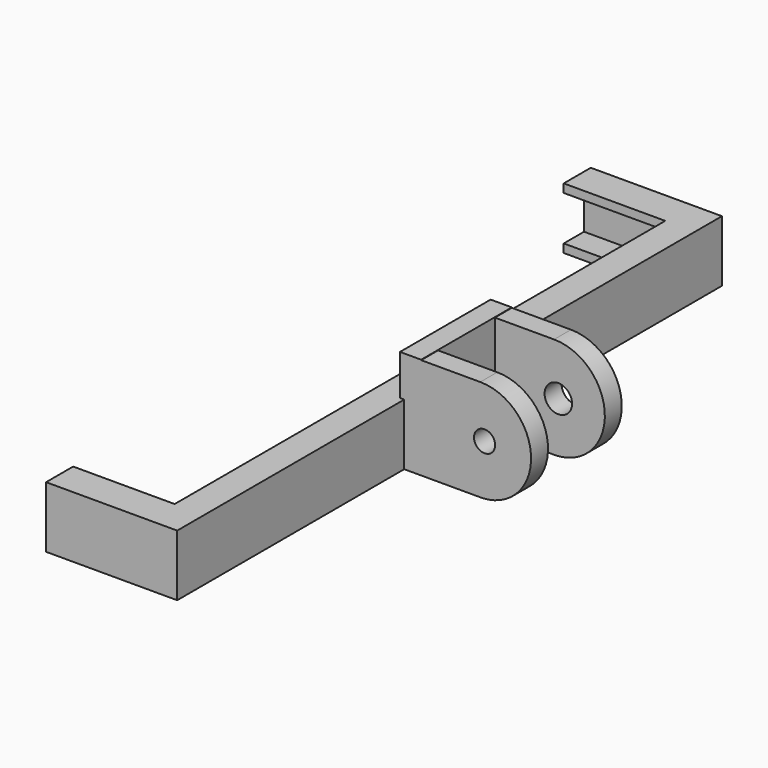
from build123d import *

# Parameters (mm, degrees)
F0_R          = 3.3
F0_R_2        = 2.5
F1_DEPTH      = 5
F2_DEPTH      = 5
F2_DEPTH_BACK = 21.8
F5_R          = 3.25
F5_R_2        = 2.5
F6_DEPTH      = 6
F7_W          = 59.1
F7_H          = 2
F7_W_2        = 6
F8_DEPTH      = 1
F7_W_3        = 13.4
F9_DEPTH      = 6
F10_DEPTH     = 30
F11_R         = 2


with BuildPart() as f1:
    # F0 (on Front) → F1 (new body)
    with BuildSketch(Plane.XZ):
        with BuildLine():
            Line((13.9969279973, 24), (0, 24))
            Line((0, 24), (0, 0))
            Line((0, 0), (14.3809281676, 0))
            ThreePointArc((14.3809281676, 0), (25.9984639003, 12.1889526569), (13.9969279973, 24))
        make_face()
        with Locations((15, 11.9969279973)):
            Circle(F0_R, mode=Mode.SUBTRACT)
        with Locations((15, 11.9969279973)):
            Circle(F0_R)
        with Locations((15, 11.9969279973)):
            Circle(F0_R_2, mode=Mode.SUBTRACT)
    extrude(amount=F1_DEPTH)

    # F0 (on Front) → F2 (join, two sides)
    with BuildSketch(Plane.XZ) as f2_sk:
        Polygon((0, 0), (0, 24), (0, 24.0955166519), (-5, 24.0955166519), (-5, 0), align=None)
    extrude(amount=F2_DEPTH)
    extrude(f2_sk.sketch, amount=-F2_DEPTH_BACK)

    # F4: F1 across plane


with BuildPart() as f1_1:
    add(f1.part)
    add(f1.part.mirror(Plane.XZ.offset(-8.4)))

    # F5 (on face) → F6 (cut)
    with BuildSketch(Plane(origin=(0, 21.8, 0), x_dir=(-1, 0, 0), z_dir=(0, 1, 0))):
        with Locations((-15, 11.9969279973)):
            Circle(F5_R)
        with Locations((-15, 11.9969279973)):
            Circle(F5_R_2, mode=Mode.SUBTRACT)
    extrude(amount=-F6_DEPTH, mode=Mode.SUBTRACT)

    # F7 (on face) → F8 (join)
    with BuildSketch(Plane(origin=(-5, 0, 0), x_dir=(0, -1, 0), z_dir=(-1, 0, 0))):
        with Locations((-51.35, 1)):
            Rectangle(F7_W, F7_H)
        with Locations((34.55, 1)):
            Rectangle(F7_W, F7_H)
        Polygon((-86.9, 0), (-80.9, 0), (-80.9, 2), (-86.9, 2), (-86.9, 1), align=None)
        Polygon((-80.9, 2), (-21.8, 2), (-21.8, 7.25), (-86.9, 7.25), (-86.9, 2), align=None)
        Polygon((5, 12.5), (5, 2), (64.1, 2), (70.1, 2), (70.1, 7.25), (70.1, 12.5), (64.1, 12.5), align=None)
        Polygon((64.1, 2), (64.1, 0), (70.1, 0), (72.1, 0), (72.1, 7.25), (72.1, 14.5), (70.1, 14.5), (70.1, 12.5), (70.1, 7.25), (70.1, 2), align=None)
        Polygon((-88.9, 0), (-86.9, 0), (-86.9, 1), (-86.9, 2), (-86.9, 7.25), (-88.9, 7.25), align=None)
        Polygon((-86.9, 7.25), (-21.8, 7.25), (-21.8, 12.5), (-80.9, 12.5), (-86.9, 12.5), align=None)
        with Locations((34.55, 13.5)):
            Rectangle(F7_W, F7_H)
        Polygon((-88.9, 7.25), (-86.9, 7.25), (-86.9, 12.5), (-86.9, 14.5), (-88.9, 14.5), align=None)
        with Locations((-51.35, 13.5)):
            Rectangle(F7_W, F7_H)
        with Locations((67.1, 13.5)):
            Rectangle(F7_W_2, F7_H)
        with Locations((-83.9, 13.5)):
            Rectangle(F7_W_2, F7_H)
    extrude(amount=-F8_DEPTH)

    # F7 (on face) → F9 (join)
    with BuildSketch(Plane(origin=(-5, 0, 0), x_dir=(0, -1, 0), z_dir=(-1, 0, 0))):
        with Locations((34.55, 13.5)):
            Rectangle(F7_W, F7_H)
        with Locations((67.1, 13.5)):
            Rectangle(F7_W_2, F7_H)
        Polygon((64.1, 2), (64.1, 0), (70.1, 0), (72.1, 0), (72.1, 7.25), (72.1, 14.5), (70.1, 14.5), (70.1, 12.5), (70.1, 7.25), (70.1, 2), align=None)
        with Locations((34.55, 1)):
            Rectangle(F7_W, F7_H)
        with Locations((-15.1, 1)):
            Rectangle(F7_W_3, F7_H)
        with Locations((-1.7, 1)):
            Rectangle(F7_W_3, F7_H)
        Polygon((-8.4, 12.5), (5, 12.5), (5, 14.5), (-8.4, 14.5), (-21.8, 14.5), (-21.8, 12.5), align=None)
        with Locations((-51.35, 13.5)):
            Rectangle(F7_W, F7_H)
        with Locations((-51.35, 1)):
            Rectangle(F7_W, F7_H)
        with Locations((-83.9, 13.5)):
            Rectangle(F7_W_2, F7_H)
        Polygon((-88.9, 7.25), (-86.9, 7.25), (-86.9, 12.5), (-86.9, 14.5), (-88.9, 14.5), align=None)
        Polygon((-88.9, 0), (-86.9, 0), (-86.9, 1), (-86.9, 2), (-86.9, 7.25), (-88.9, 7.25), align=None)
        Polygon((-86.9, 0), (-80.9, 0), (-80.9, 2), (-86.9, 2), (-86.9, 1), align=None)
    extrude(amount=F9_DEPTH)

    # F7 (on face) → F10 (join)
    with BuildSketch(Plane(origin=(-5, 0, 0), x_dir=(0, -1, 0), z_dir=(-1, 0, 0))):
        with Locations((-83.9, 13.5)):
            Rectangle(F7_W_2, F7_H)
        Polygon((-88.9, 7.25), (-86.9, 7.25), (-86.9, 12.5), (-86.9, 14.5), (-88.9, 14.5), align=None)
        Polygon((-88.9, 0), (-86.9, 0), (-86.9, 1), (-86.9, 2), (-86.9, 7.25), (-88.9, 7.25), align=None)
        Polygon((-86.9, 0), (-80.9, 0), (-80.9, 2), (-86.9, 2), (-86.9, 1), align=None)
        Polygon((64.1, 2), (64.1, 0), (70.1, 0), (72.1, 0), (72.1, 7.25), (72.1, 14.5), (70.1, 14.5), (70.1, 12.5), (70.1, 7.25), (70.1, 2), align=None)
        with Locations((67.1, 13.5)):
            Rectangle(F7_W_2, F7_H)
    extrude(amount=F10_DEPTH)

    # F11
    f11_edges = [f1_1.edges().sort_by_distance(p)[0] for p in [
        (-20, -70.1, 12.5),
        (-5, 8.4, 12.5),
        (-20, 86.9, 12.5),
    ]]
    fillet(f11_edges, radius=F11_R)


solid = f1_1.part
